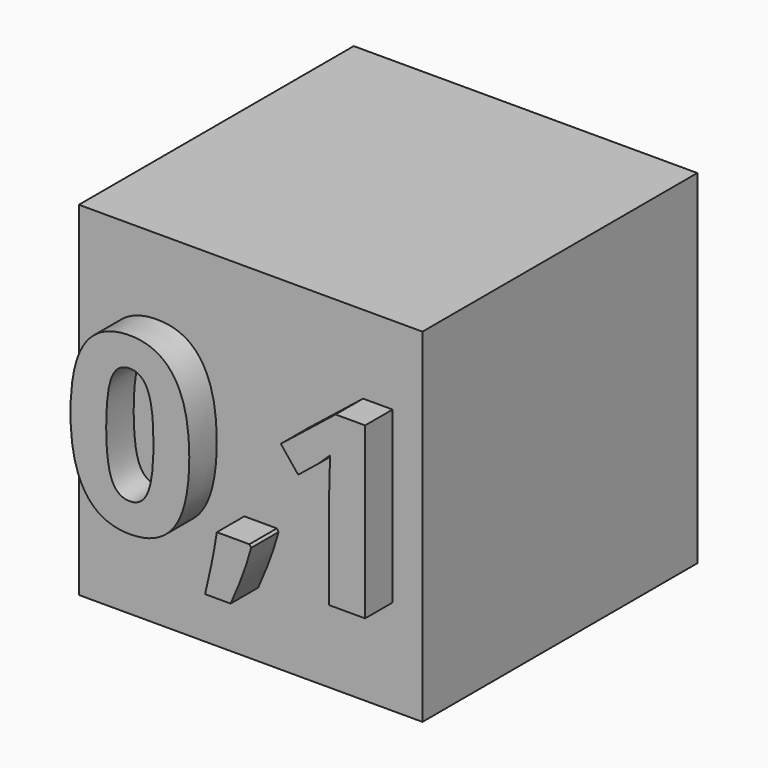
from build123d import *

# Parameters (mm, degrees)
F0_W         = 20
F0_H         = 20
F1_DEPTH     = 20
F2_TEXT_SIZE = 13.8551320156
F3_DEPTH     = 2


# Not quite as in the source:
# - Text() gives the source's letters only with a copy of the font that has no kerning and outlines rounded to 1/6400 em; it was checked with that copy


with BuildPart() as f1:
    # F0 (on Front) → F1 (new body)
    with BuildSketch(Plane.XZ):
        with Locations((-10, 10)):
            Rectangle(F0_W, F0_H)
    extrude(amount=F1_DEPTH)

    # F2 (on face) → F3 (join)
    with BuildSketch(Plane.XZ.offset(20)):
        with Locations((-19.3889588118, 5.5522602051)):
            Text('0,1', F2_TEXT_SIZE, font='Open Sans', font_style=FontStyle.BOLD, text_align=(TextAlign.LEFT, TextAlign.BOTTOM))
    extrude(amount=F3_DEPTH)


solid = f1.part
